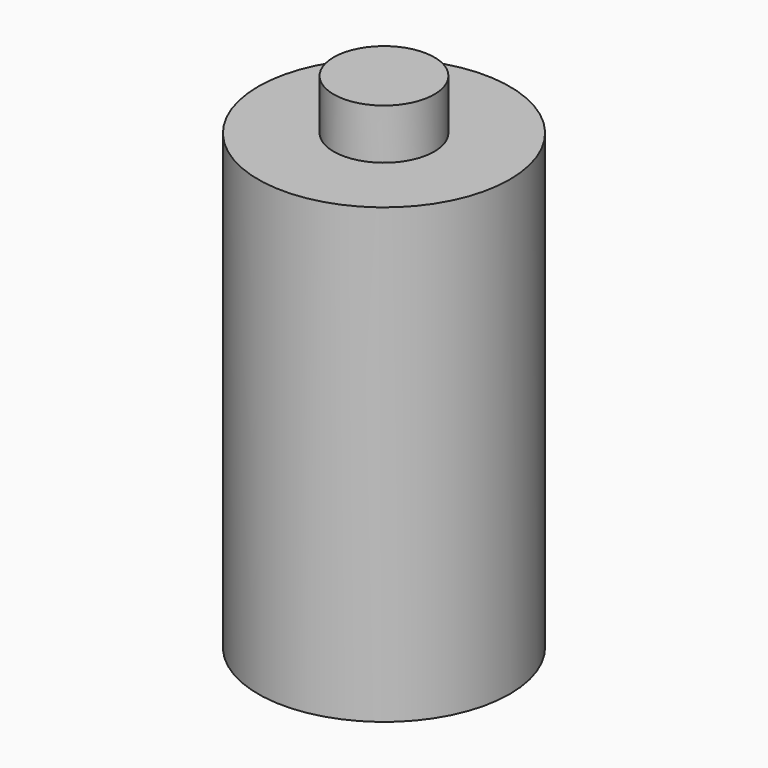
from build123d import *


# Not quite as in the source:
# - the program builds the solid bodies; features that only make, move or delete a surface that nothing else refers to are left out


with BuildPart() as f1:
    # F0 (on Front) → F1 (revolve)
    with BuildSketch(Plane.XZ):
        Polygon((0, -34.307694056), (0, 65.692305944), (-10, 65.692305944), (-10, 55.692305944), (-25, 55.692305944), (-25, -34.307694056), align=None)
    revolve(axis=Axis((0, 0, 15.692305944), (0, 0, 1)))


solid = f1.part
